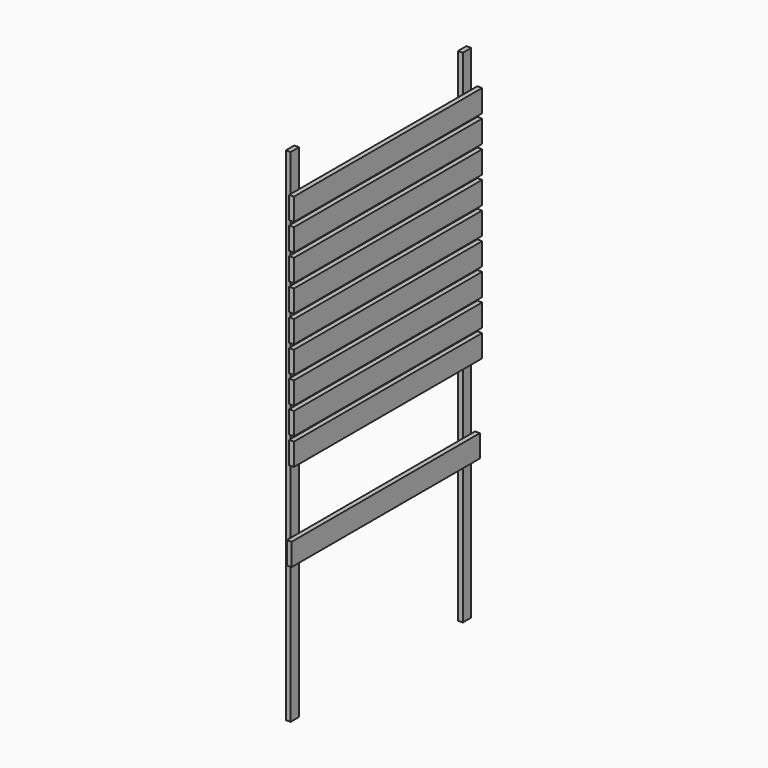
from build123d import *

# Parameters (mm, degrees)
F0_W     = 19
F0_H     = 42
F1_DEPTH = 89
F2_DEPTH = 557
F3_DEPTH = 2000
F4_W     = 469
F4_H     = 89
F5_DEPTH = 19


# Not quite as in the source:
# - a feature names something its author has since deleted; it is built from what else it names


with BuildPart() as f1:
    # F0 (on Top) → F1 (new body)
    with BuildSketch(Plane.XY):
        Polygon((-9.5, -469), (9.5, -469), (9.5, 469), (-9.5, 469), (-9.5, 450), (-9.5, 408), (-9.5, -408), (-9.5, -450), align=None)
        with Locations((-19, -429)):
            Rectangle(F0_W, F0_H)
        with Locations((-19, 429)):
            Rectangle(F0_W, F0_H)
    extrude(amount=F1_DEPTH)

    # F0 (on Top) → F2 (join)
    with BuildSketch(Plane.XY):
        with Locations((-19, -429)):
            Rectangle(F0_W, F0_H)
        with Locations((-19, 429)):
            Rectangle(F0_W, F0_H)
    extrude(amount=-F2_DEPTH)

    # F3 (add): faces of the model
    f3_faces = [f1.faces().sort_by_distance(p)[0] for p in [
        (-19, 429, -557),
        (-19, -429, -557),
    ]]
    extrude(f3_faces, amount=-F3_DEPTH)


with BuildPart() as f5:
    # F4 (on Right) → F5 (new body)
    with BuildSketch(Plane.YZ):
        Polygon((64.7416710854, 443.7016204007), (0, 443.7016204007), (0, 354.7016204007), (469, 354.7016204007), (469, 443.7016204007), align=None)
        with Locations((-234.5, 399.2016204007)):
            Rectangle(F4_W, F4_H)
    extrude(amount=F5_DEPTH)


with BuildPart() as f5b:
    # F4 (on Right) → F5, piece 2 (new body)
    with BuildSketch(Plane.YZ):
        Polygon((51.5239238739, 551.2016204007), (0, 551.2016204007), (0, 462.2016204007), (64.7416710854, 462.2016204007), (469, 462.2016204007), (469, 551.2016204007), align=None)
        with Locations((-234.5, 506.7016204007)):
            Rectangle(F4_W, F4_H)
    extrude(amount=F5_DEPTH)


with BuildPart() as f5c:
    # F4 (on Right) → F5, piece 3 (new body)
    with BuildSketch(Plane.YZ):
        Polygon((59.0889453888, 658.7016204007), (0, 658.7016204007), (0, 569.7016204007), (51.5239238739, 569.7016204007), (469, 569.7016204007), (469, 658.7016204007), align=None)
        with Locations((-234.5, 614.2016204007)):
            Rectangle(F4_W, F4_H)
    extrude(amount=F5_DEPTH)


with BuildPart() as f5d:
    # F4 (on Right) → F5, piece 4 (new body)
    with BuildSketch(Plane.YZ):
        with Locations((-234.5, 1259.2016204007)):
            Rectangle(F4_W, F4_H)
        Polygon((0, 1303.7016204007), (0, 1214.7016204007), (46.117246151, 1214.7016204007), (469, 1214.7016204007), (469, 1303.7016204007), align=None)
    extrude(amount=F5_DEPTH)


with BuildPart() as f5e:
    # F4 (on Right) → F5, piece 5 (new body)
    with BuildSketch(Plane.YZ):
        with Locations((-234.5, 1151.7016204007)):
            Rectangle(F4_W, F4_H)
        Polygon((0, 1196.2016204007), (0, 1107.2016204007), (34.1612100601, 1107.2016204007), (469, 1107.2016204007), (469, 1196.2016204007), (46.117246151, 1196.2016204007), align=None)
    extrude(amount=F5_DEPTH)


with BuildPart() as f5f:
    # F4 (on Right) → F5, piece 6 (new body)
    with BuildSketch(Plane.YZ):
        with Locations((-234.5, 1044.2016204007)):
            Rectangle(F4_W, F4_H)
        Polygon((0, 1088.7016204007), (0, 999.7016204007), (44.2955195904, 999.7016204007), (469, 999.7016204007), (469, 1088.7016204007), (34.1612100601, 1088.7016204007), align=None)
    extrude(amount=F5_DEPTH)


with BuildPart() as f5g:
    # F4 (on Right) → F5, piece 7 (new body)
    with BuildSketch(Plane.YZ):
        with Locations((-234.5, 936.7016204007)):
            Rectangle(F4_W, F4_H)
        Polygon((0, 981.2016204007), (0, 892.2016204007), (57.986497879, 892.2016204007), (469, 892.2016204007), (469, 981.2016204007), (44.2955195904, 981.2016204007), align=None)
    extrude(amount=F5_DEPTH)


with BuildPart() as f5h:
    # F4 (on Right) → F5, piece 8 (new body)
    with BuildSketch(Plane.YZ):
        with Locations((-234.5, 829.2016204007)):
            Rectangle(F4_W, F4_H)
        Polygon((0, 873.7016204007), (0, 784.7016204007), (90.5175209045, 784.7016204007), (469, 784.7016204007), (469, 873.7016204007), (57.986497879, 873.7016204007), align=None)
    extrude(amount=F5_DEPTH)


with BuildPart() as f5i:
    # F4 (on Right) → F5, piece 9 (new body)
    with BuildSketch(Plane.YZ):
        with Locations((-234.5, 721.7016204007)):
            Rectangle(F4_W, F4_H)
        Polygon((0, 766.2016204007), (0, 677.2016204007), (59.0889453888, 677.2016204007), (469, 677.2016204007), (469, 766.2016204007), (90.5175209045, 766.2016204007), align=None)
    extrude(amount=F5_DEPTH)


solid = Compound([f1.part, f5.part, f5b.part, f5c.part, f5d.part, f5e.part, f5f.part, f5g.part, f5h.part, f5i.part])
